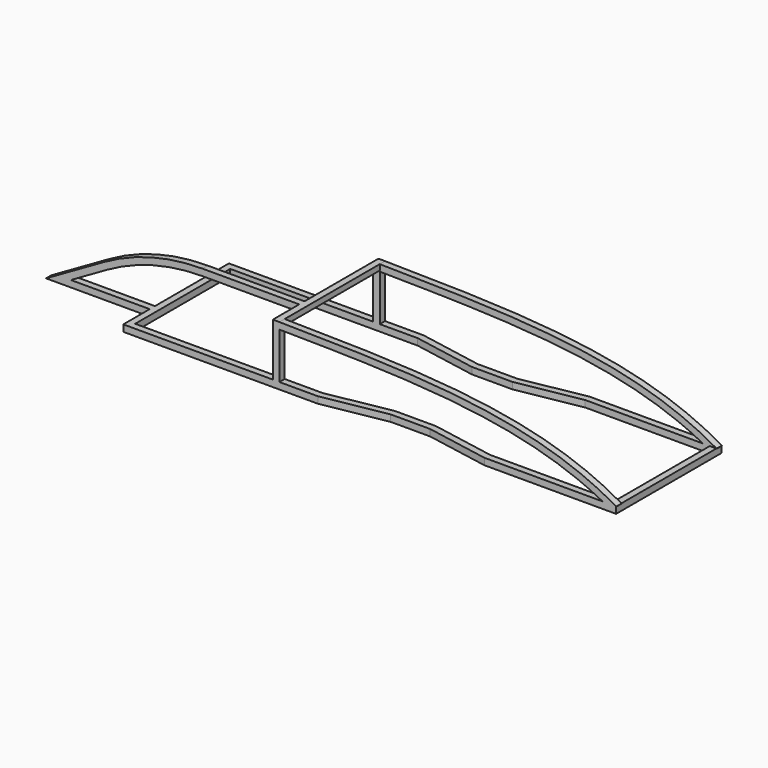
from build123d import *

# Parameters (mm, degrees)
F0_W     = 20
F0_H     = 20
F1_DEPTH = 20
F2_DEPTH = 180
F3_W     = 20
F3_H     = 16.9352668524
F4_DEPTH = 360
F6_START = -280
F6_DEPTH = 20
F7_DEPTH = 20
F8_START = -380
F8_DEPTH = 20


# Not quite as in the source:
# - the dataset's text gives a spline's control points without its knots; the knots are read off the source's solid


with BuildPart() as f1:
    # F0 (on Top) → F1 (new body)
    with BuildSketch(Plane.XY):
        Polygon((-726.5, -180), (-726.5, 180), (-293.5, 180), (-293.5, 200), (-746.5, 200), (-746.5, -200), (-293.5, -200), (-293.5, -180), align=None)
        with Locations((-283.5, 190)):
            Rectangle(F0_W, F0_H)
        Polygon((-273.5, 200), (-273.5, 180), (-158.6148713515, 180), (33.3502043798, 145), (95.158547163, 145), (156.9668899462, 145), (348.9319656775, 180), (726.5, 180), (726.5, -180), (348.9319656775, -180), (156.9668899462, -145), (95.158547163, -145), (33.3502043798, -145), (-158.6148713515, -180), (-273.5, -180), (-273.5, -200), (-156.8065285683, -200), (35.158547163, -165), (95.158547163, -165), (155.158547163, -165), (347.1236228943, -200), (746.5, -200), (746.5, 200), (347.1236228943, 200), (155.158547163, 165), (95.158547163, 165), (35.158547163, 165), (-156.8065285683, 200), align=None)
        with Locations((-283.5, -190)):
            Rectangle(F0_W, F0_H)
    extrude(amount=F1_DEPTH)

    # F0 (on Top) → F2 (join)
    with BuildSketch(Plane.XY):
        with Locations((-283.5, 190)):
            Rectangle(F0_W, F0_H)
        with Locations((-283.5, -190)):
            Rectangle(F0_W, F0_H)
    extrude(amount=F2_DEPTH)

    # F3 (on face) → F4 (join, through all)
    with BuildSketch(Plane.XZ.offset(-180)):
        with Locations((-283.5, 171.5323665738)):
            Rectangle(F3_W, F3_H)
    extrude(amount=F4_DEPTH)

    # F5 (on face) → F6 (join)
    with BuildSketch(Plane(origin=(0, 200, 0), x_dir=(-1, 0, 0), z_dir=(0, 1, 0)).offset(F6_START)):
        with BuildLine():
            Line((586.6939193795, 180), (293.5, 180))
            Line((293.5, 180), (293.5, 160))
            Line((293.5, 160), (586.6939193795, 160))
            ThreePointArc((586.6939193795, 160), (735.9691353026, 140.4613366782), (875.1869781698, 83.1617583142))
            Line((875.1869781698, 83.1617583142), (985.3476229522, 20))
            Line((985.3476229522, 20), (746.5, 20))
            Line((746.5, 20), (746.5, 0))
            Line((746.5, 0), (1060.4386329651, 0))
            Line((1060.4386329651, 0), (885.1350146798, 100.5121637733))
            ThreePointArc((885.1350146798, 100.5121637733), (741.1165565413, 159.7875896671), (586.6939193795, 180))
        make_face()
    extrude(amount=-F6_DEPTH)

    # F5 (on face) → F7 (join)
    with BuildSketch(Plane(origin=(0, 200, 0), x_dir=(-1, 0, 0), z_dir=(0, 1, 0))):
        with BuildLine():
            Line((273.5, 159.9987796237), (273.5, 180))
            add(Edge.make_bspline(
                [(273.5, 180), (-155.7328006583, 175.2587886422), (-491.770210992, 167.9634028537), (-747.1652626991, 20)],
                knots=[0, 0, 0, 0, 1033.1299910857, 1033.1299910857, 1033.1299910857, 1033.1299910857], degree=3))
            Line((-747.1652626991, 20), (-737.139304978, 2.6945045788))
            add(Edge.make_bspline(
                [(273.5, 159.9987796237), (166.3014372689, 158.8143761406), (14.3965034251, 156.7944993715), (-170.7291731338, 147.1968180223), (-300.9944872791, 134.9583970227), (-422.7375996574, 116.1215761349), (-536.0847045329, 89.1569939237), (-641.215968445, 52.559680727), (-706.007134323, 20.7309617362), (-737.139304978, 2.6945045788)],
                knots=[0.0001715991, 0.0001715991, 0.0001715991, 0.0001715991, 0.25, 0.375, 0.5, 0.625, 0.75, 0.875, 1, 1, 1, 1], degree=3))
        make_face()
    extrude(amount=-F7_DEPTH)

    # F5 (on face) → F8 (join)
    with BuildSketch(Plane(origin=(0, 200, 0), x_dir=(-1, 0, 0), z_dir=(0, 1, 0)).offset(F8_START)):
        with BuildLine():
            Line((273.5, 159.9987796237), (273.5, 180))
            add(Edge.make_bspline(
                [(273.5, 180), (-155.7328006583, 175.2587886422), (-491.770210992, 167.9634028537), (-747.1652626991, 20)],
                knots=[0, 0, 0, 0, 1033.1299910857, 1033.1299910857, 1033.1299910857, 1033.1299910857], degree=3))
            Line((-747.1652626991, 20), (-737.139304978, 2.6945045788))
            add(Edge.make_bspline(
                [(273.5, 159.9987796237), (166.3014372689, 158.8143761406), (14.3965034251, 156.7944993715), (-170.7291731338, 147.1968180223), (-300.9944872791, 134.9583970227), (-422.7375996574, 116.1215761349), (-536.0847045329, 89.1569939237), (-641.215968445, 52.559680727), (-706.007134323, 20.7309617362), (-737.139304978, 2.6945045788)],
                knots=[0.0001715991, 0.0001715991, 0.0001715991, 0.0001715991, 0.25, 0.375, 0.5, 0.625, 0.75, 0.875, 1, 1, 1, 1], degree=3))
        make_face()
    extrude(amount=-F8_DEPTH)


solid = f1.part
